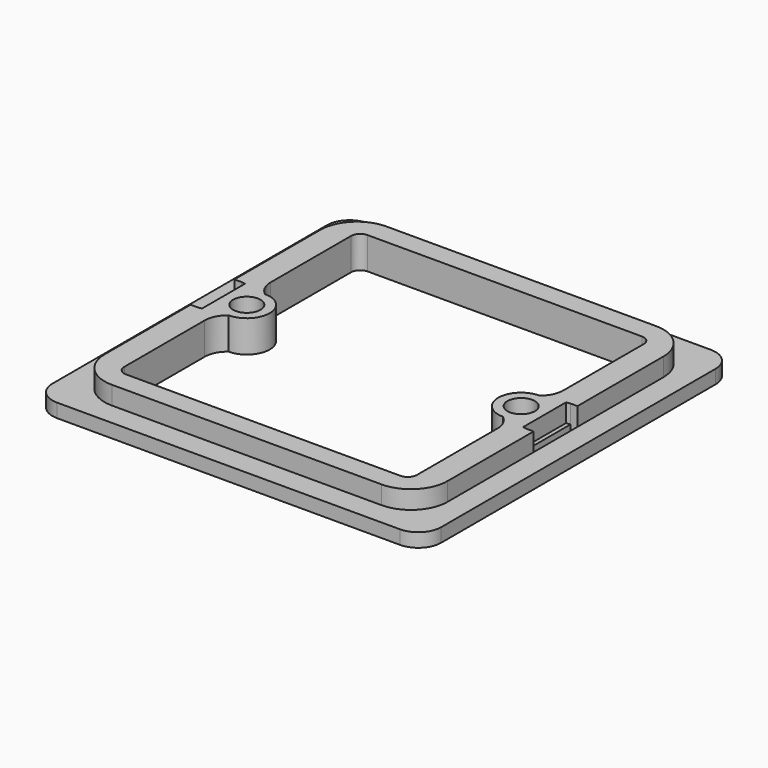
from build123d import *

# Parameters (mm, degrees)
F0_W        = 85
F0_H        = 85
F1_DEPTH    = 3
F2_R        = 5
F3_DEPTH    = 7
F4_R        = 8
F5_R        = 2
F6_T1_DEPTH = 7


# Not quite as in the source:
# - a fillet or chamfer that OpenCascade refuses, or shapes differently, is made with other operations: its cross-section is extruded or revolved along the edge and cut away or added


with BuildPart() as f1:
    # F0 (on Top) → F1 (new body)
    with BuildSketch(Plane.XY):
        Rectangle(F0_W, F0_H)
        Polygon((-37.5, -6), (-37.5, 6), (-37.5, 37.5), (37.5, 37.5), (37.5, 6), (37.5, -6), (37.5, -37.5), (-37.5, -37.5), align=None, mode=Mode.SUBTRACT)
        Polygon((-35.1, -35.1), (-35.1, -5.85), (-36, -6), (-37.5, -6), (-37.5, -37.5), (37.5, -37.5), (37.5, -6), (36, -6), (35.1, -5.85), (35.1, -35.1), align=None)
        Polygon((-36, 6), (-35.1, 5.85), (-35.1, 35.1), (35.1, 35.1), (35.1, 5.85), (36, 6), (37.5, 6), (37.5, 37.5), (-37.5, 37.5), (-37.5, 6), align=None)
        Polygon((-32, 5.3333333333), (-32, 33), (32, 33), (32, 5.3333333333), (35.1, 5.85), (35.1, 35.1), (-35.1, 35.1), (-35.1, 5.85), align=None)
        with BuildLine():
            Line((-32, 4.582575695), (-32, 5.3333333333))
            Line((-32, 5.3333333333), (-35.1, 5.85))
            Line((-35.1, 5.85), (-35.1, -5.85))
            Line((-35.1, -5.85), (-32, -5.3333333333))
            Line((-32, -5.3333333333), (-32, -4.582575695))
            ThreePointArc((-32, -4.582575695), (-35, 0), (-32, 4.582575695))
        make_face()
        Polygon((-35.1, -5.85), (-35.1, 5.85), (-36, 6), (-36, -6), align=None)
        with BuildLine():
            ThreePointArc((-30, 5), (-31.0215482184, 4.8945315647), (-32, 4.582575695))
            Line((-32, 4.582575695), (-32, 2.2360679775))
            ThreePointArc((-32, 2.2360679775), (-28.7752551286, 2.7386127875), (-27, 0))
            ThreePointArc((-27, 0), (-28.7752551286, -2.7386127875), (-32, -2.2360679775))
            Line((-32, -2.2360679775), (-32, -4.582575695))
            ThreePointArc((-32, -4.582575695), (-31.0215482184, -4.8945315647), (-30, -5))
            ThreePointArc((-30, -5), (-26.4644660941, -3.5355339059), (-25, 0))
            ThreePointArc((-25, 0), (-26.4644660941, 3.5355339059), (-30, 5))
        make_face()
        with BuildLine():
            Line((-30, 5), (-32, 5.3333333333))
            Line((-32, 5.3333333333), (-32, 4.582575695))
            ThreePointArc((-32, 4.582575695), (-31.0215482184, 4.8945315647), (-30, 5))
        make_face()
        with BuildLine():
            ThreePointArc((-30, -5), (-31.0215482184, -4.8945315647), (-32, -4.582575695))
            Line((-32, -4.582575695), (-32, -5.3333333333))
            Line((-32, -5.3333333333), (-30, -5))
        make_face()
        Polygon((-32, -5.3333333333), (-35.1, -5.85), (-35.1, -35.1), (35.1, -35.1), (35.1, -5.85), (32, -5.3333333333), (32, -33), (-32, -33), align=None)
        with BuildLine():
            Line((35.1, 5.85), (32, 5.3333333333))
            Line((32, 5.3333333333), (32, 4.582575695))
            ThreePointArc((32, 4.582575695), (34.1833001327, 2.7386127875), (35, 0))
            ThreePointArc((35, 0), (34.1833001327, -2.7386127875), (32, -4.582575695))
            Line((32, -4.582575695), (32, -5.3333333333))
            Line((32, -5.3333333333), (35.1, -5.85))
            Line((35.1, -5.85), (35.1, 5.85))
        make_face()
        with BuildLine():
            Line((32, 4.582575695), (32, 5.3333333333))
            Line((32, 5.3333333333), (30, 5))
            ThreePointArc((30, 5), (31.0215482184, 4.8945315647), (32, 4.582575695))
        make_face()
        with BuildLine():
            ThreePointArc((32, -4.582575695), (31.0215482184, -4.8945315647), (30, -5))
            Line((30, -5), (32, -5.3333333333))
            Line((32, -5.3333333333), (32, -4.582575695))
        make_face()
        with BuildLine():
            Line((32, 2.2360679775), (32, 4.582575695))
            ThreePointArc((32, 4.582575695), (31.0215482184, 4.8945315647), (30, 5))
            ThreePointArc((30, 5), (25, 0), (30, -5))
            ThreePointArc((30, -5), (31.0215482184, -4.8945315647), (32, -4.582575695))
            Line((32, -4.582575695), (32, -2.2360679775))
            ThreePointArc((32, -2.2360679775), (27, 0), (32, 2.2360679775))
        make_face()
        with BuildLine():
            ThreePointArc((35, 0), (34.1833001327, 2.7386127875), (32, 4.582575695))
            Line((32, 4.582575695), (32, 2.2360679775))
            ThreePointArc((32, 2.2360679775), (32.7386127875, 1.2247448714), (33, 0))
            ThreePointArc((33, 0), (32.7386127875, -1.2247448714), (32, -2.2360679775))
            Line((32, -2.2360679775), (32, -4.582575695))
            ThreePointArc((32, -4.582575695), (34.1833001327, -2.7386127875), (35, 0))
        make_face()
        with BuildLine():
            Line((-32, 2.2360679775), (-32, 4.582575695))
            ThreePointArc((-32, 4.582575695), (-35, 0), (-32, -4.582575695))
            Line((-32, -4.582575695), (-32, -2.2360679775))
            ThreePointArc((-32, -2.2360679775), (-33, 0), (-32, 2.2360679775))
        make_face()
        Polygon((36, 6), (35.1, 5.85), (35.1, -5.85), (36, -6), align=None)
    extrude(amount=F1_DEPTH)

    # F2
    f2_edges = [f1.edges().sort_by_distance(p)[0] for p in [
        (-42.5, 42.5, 1.5),
        (-42.5, -42.5, 1.5),
        (42.5, -42.5, 1.5),
        (42.5, 42.5, 1.5),
    ]]
    fillet(f2_edges, radius=F2_R)

    # F0 (on Top) → F3 (join)
    with BuildSketch(Plane.XY):
        with BuildLine():
            Line((-32, 4.582575695), (-32, 5.3333333333))
            Line((-32, 5.3333333333), (-35.1, 5.85))
            Line((-35.1, 5.85), (-35.1, -5.85))
            Line((-35.1, -5.85), (-32, -5.3333333333))
            Line((-32, -5.3333333333), (-32, -4.582575695))
            ThreePointArc((-32, -4.582575695), (-35, 0), (-32, 4.582575695))
        make_face()
        with BuildLine():
            Line((-30, 5), (-32, 5.3333333333))
            Line((-32, 5.3333333333), (-32, 4.582575695))
            ThreePointArc((-32, 4.582575695), (-31.0215482184, 4.8945315647), (-30, 5))
        make_face()
        with BuildLine():
            ThreePointArc((-30, 5), (-31.0215482184, 4.8945315647), (-32, 4.582575695))
            Line((-32, 4.582575695), (-32, 2.2360679775))
            ThreePointArc((-32, 2.2360679775), (-28.7752551286, 2.7386127875), (-27, 0))
            ThreePointArc((-27, 0), (-28.7752551286, -2.7386127875), (-32, -2.2360679775))
            Line((-32, -2.2360679775), (-32, -4.582575695))
            ThreePointArc((-32, -4.582575695), (-31.0215482184, -4.8945315647), (-30, -5))
            ThreePointArc((-30, -5), (-26.4644660941, -3.5355339059), (-25, 0))
            ThreePointArc((-25, 0), (-26.4644660941, 3.5355339059), (-30, 5))
        make_face()
        with BuildLine():
            Line((-32, 2.2360679775), (-32, 4.582575695))
            ThreePointArc((-32, 4.582575695), (-35, 0), (-32, -4.582575695))
            Line((-32, -4.582575695), (-32, -2.2360679775))
            ThreePointArc((-32, -2.2360679775), (-33, 0), (-32, 2.2360679775))
        make_face()
        with BuildLine():
            ThreePointArc((-30, -5), (-31.0215482184, -4.8945315647), (-32, -4.582575695))
            Line((-32, -4.582575695), (-32, -5.3333333333))
            Line((-32, -5.3333333333), (-30, -5))
        make_face()
        Polygon((-32, -5.3333333333), (-35.1, -5.85), (-35.1, -35.1), (35.1, -35.1), (35.1, -5.85), (32, -5.3333333333), (32, -33), (-32, -33), align=None)
        Polygon((-35.1, -35.1), (-35.1, -5.85), (-36, -6), (-37.5, -6), (-37.5, -37.5), (37.5, -37.5), (37.5, -6), (36, -6), (35.1, -5.85), (35.1, -35.1), align=None)
        Polygon((-36, 6), (-35.1, 5.85), (-35.1, 35.1), (35.1, 35.1), (35.1, 5.85), (36, 6), (37.5, 6), (37.5, 37.5), (-37.5, 37.5), (-37.5, 6), align=None)
        Polygon((-32, 5.3333333333), (-32, 33), (32, 33), (32, 5.3333333333), (35.1, 5.85), (35.1, 35.1), (-35.1, 35.1), (-35.1, 5.85), align=None)
        with BuildLine():
            ThreePointArc((32, -4.582575695), (31.0215482184, -4.8945315647), (30, -5))
            Line((30, -5), (32, -5.3333333333))
            Line((32, -5.3333333333), (32, -4.582575695))
        make_face()
        with BuildLine():
            Line((32, 2.2360679775), (32, 4.582575695))
            ThreePointArc((32, 4.582575695), (31.0215482184, 4.8945315647), (30, 5))
            ThreePointArc((30, 5), (25, 0), (30, -5))
            ThreePointArc((30, -5), (31.0215482184, -4.8945315647), (32, -4.582575695))
            Line((32, -4.582575695), (32, -2.2360679775))
            ThreePointArc((32, -2.2360679775), (27, 0), (32, 2.2360679775))
        make_face()
        with BuildLine():
            Line((32, 4.582575695), (32, 5.3333333333))
            Line((32, 5.3333333333), (30, 5))
            ThreePointArc((30, 5), (31.0215482184, 4.8945315647), (32, 4.582575695))
        make_face()
        with BuildLine():
            ThreePointArc((35, 0), (34.1833001327, 2.7386127875), (32, 4.582575695))
            Line((32, 4.582575695), (32, 2.2360679775))
            ThreePointArc((32, 2.2360679775), (32.7386127875, 1.2247448714), (33, 0))
            ThreePointArc((33, 0), (32.7386127875, -1.2247448714), (32, -2.2360679775))
            Line((32, -2.2360679775), (32, -4.582575695))
            ThreePointArc((32, -4.582575695), (34.1833001327, -2.7386127875), (35, 0))
        make_face()
        with BuildLine():
            Line((35.1, 5.85), (32, 5.3333333333))
            Line((32, 5.3333333333), (32, 4.582575695))
            ThreePointArc((32, 4.582575695), (34.1833001327, 2.7386127875), (35, 0))
            ThreePointArc((35, 0), (34.1833001327, -2.7386127875), (32, -4.582575695))
            Line((32, -4.582575695), (32, -5.3333333333))
            Line((32, -5.3333333333), (35.1, -5.85))
            Line((35.1, -5.85), (35.1, 5.85))
        make_face()
    extrude(amount=F3_DEPTH)

    # F4
    f4_edges = [f1.edges().sort_by_distance(p)[0] for p in [
        (-37.5, -37.5, 5),
        (37.5, -37.5, 5),
        (37.5, 37.5, 5),
        (-37.5, 37.5, 5),
    ]]
    fillet(f4_edges, radius=F4_R)

    # F5
    f5_edges = [f1.edges().sort_by_distance(p)[0] for p in [
        (32, -33, 3.5),
        (-32, -33, 3.5),
        (-32, 33, 3.5),
        (32, 33, 3.5),
    ]]
    fillet(f5_edges, radius=F5_R)

    # F6: fillet of radius 5 on 4 edges, made by hand

    # F6_s2 → F6_t1 (join)
    with BuildSketch(Plane.XY):
        with BuildLine():
            ThreePointArc((30, -5), (31.472135955, -6.7639320225), (32, -9))
            Line((32, -9), (32, -5.3333333333))
            Line((32, -5.3333333333), (30, -5))
        make_face()
        with BuildLine():
            ThreePointArc((32, 9), (31.472135955, 6.7639320225), (30, 5))
            Line((30, 5), (32, 5.3333333333))
            Line((32, 5.3333333333), (32, 9))
        make_face()
        with BuildLine():
            ThreePointArc((-32, 9), (-31.472135955, 6.7639320225), (-30, 5))
            Line((-30, 5), (-32, 5.3333333333))
            Line((-32, 5.3333333333), (-32, 9))
        make_face()
        with BuildLine():
            ThreePointArc((-30, -5), (-31.472135955, -6.7639320225), (-32, -9))
            Line((-32, -9), (-32, -5.3333333333))
            Line((-32, -5.3333333333), (-30, -5))
        make_face()
    extrude(amount=F6_T1_DEPTH)


solid = f1.part
